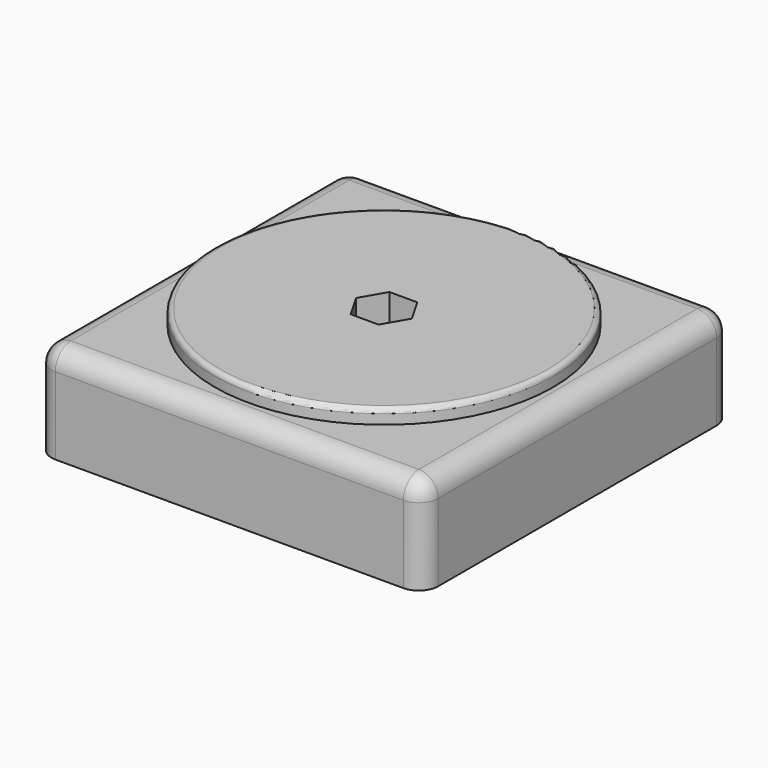
from build123d import *

# Parameters (mm, degrees)
F0_W      = 101.6
F0_H      = 101.6
F1_DEPTH  = 25.4
F2_R      = 38.1
F3_DEPTH  = 22.86
F4_R      = 37.973
F5_DEPTH  = 3.81
F6_R      = 44.45
F6_R_2    = 37.973
F7_DEPTH  = 3.81
F8_R      = 5.08
F9_R      = 1.27
F12_DEPTH = 248.92


with BuildPart() as f1:
    # F0 (on Top) → F1 (new body)
    with BuildSketch(Plane.XY):
        Rectangle(F0_W, F0_H)
    extrude(amount=F1_DEPTH)

    # F2 (on face) → F3 (cut)
    with BuildSketch(Plane.XY.offset(25.4)):
        Circle(F2_R)
    extrude(amount=-F3_DEPTH, mode=Mode.SUBTRACT)

    # F8
    f8_edges = [f1.edges().sort_by_distance(p)[0] for p in [
        (-50.8, -50.8, 12.7),
        (50.8, -50.8, 12.7),
        (50.8, 50.8, 12.7),
        (-50.8, 50.8, 12.7),
        (0, 50.8, 25.4),
        (-50.8, 0, 25.4),
        (50.8, 0, 25.4),
        (0, -50.8, 25.4),
    ]]
    fillet(f8_edges, radius=F8_R)


with BuildPart() as f5:
    # F4 (on face) → F5 (new body)
    with BuildSketch(Plane.XY.offset(25.4)):
        Circle(F4_R)
    extrude(amount=-F5_DEPTH)

    # F6 (on face) → F7 (join)
    with BuildSketch(Plane.XY.offset(25.4)):
        Circle(F6_R)
        Circle(F6_R_2, mode=Mode.SUBTRACT)
        Circle(F6_R_2)
    extrude(amount=F7_DEPTH)

    # F9
    f9_edges = [f5.edges().sort_by_distance(p)[0] for p in [
        (-44.45, 0, 29.21),
    ]]
    fillet(f9_edges, radius=F9_R)


with BuildPart() as f12:
    # F11 (on offset) → F12 (new body)
    with BuildSketch(Plane.XY.offset(127)):
        Polygon((3.6661742094, 6.35), (-3.6661742094, 6.35), (-7.3323484187, 0), (-3.6661742094, -6.35), (3.6661742094, -6.35), (7.3323484187, 0), align=None)
    extrude(amount=-F12_DEPTH)


with BuildPart() as f1_1:
    add(f1.part)

    # F13: cut F12
    add(f12.part, mode=Mode.SUBTRACT)


with BuildPart() as f5_1:
    add(f5.part)

    # F13: cut F12
    add(f12.part, mode=Mode.SUBTRACT)


solid = Compound([f1_1.part, f5_1.part])
